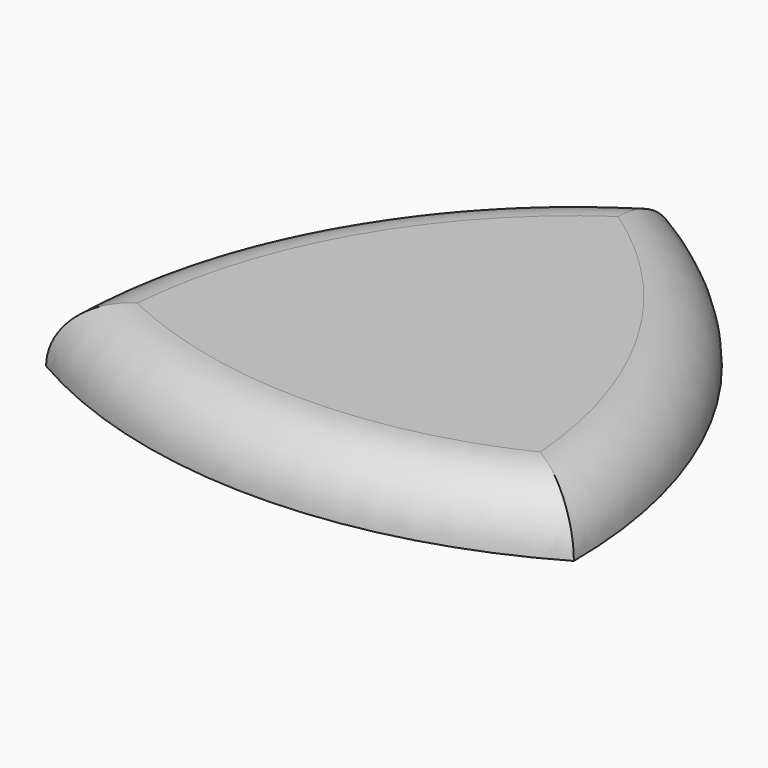
from build123d import *

# Parameters (mm, degrees)
F1_DEPTH = 5
F2_R     = 4.99999


# Not quite as in the source:
# - a fillet or chamfer is up to 0.001 mm smaller than in the source, because OpenCascade refuses the exact size
# - a feature of the source that left no trace in its solid (it failed there, or was rolled back) is left out


with BuildPart() as f1:
    # F0 (on Top) → F1 (new body)
    with BuildSketch(Plane.XY):
        with BuildLine():
            ThreePointArc((-21.6506350946, -12.5), (0, -18.3012701892), (21.6506350946, -12.5))
            ThreePointArc((21.6506350946, -12.5), (15.8493649054, 9.1506350946), (0, 25))
            ThreePointArc((0, 25), (-15.8493649054, 9.1506350946), (-21.6506350946, -12.5))
        make_face()
    extrude(amount=F1_DEPTH)

    # F2 (radius 5 in the source; OpenCascade refuses exactly that, so slightly less here)
    f2_edges = [f1.edges().sort_by_distance(p)[0] for p in [
        (-15.849365, 9.150635, 5),
        (0, -18.30127, 5),
        (15.849365, 9.150635, 5),
    ]]
    fillet(f2_edges, radius=F2_R)


solid = f1.part
